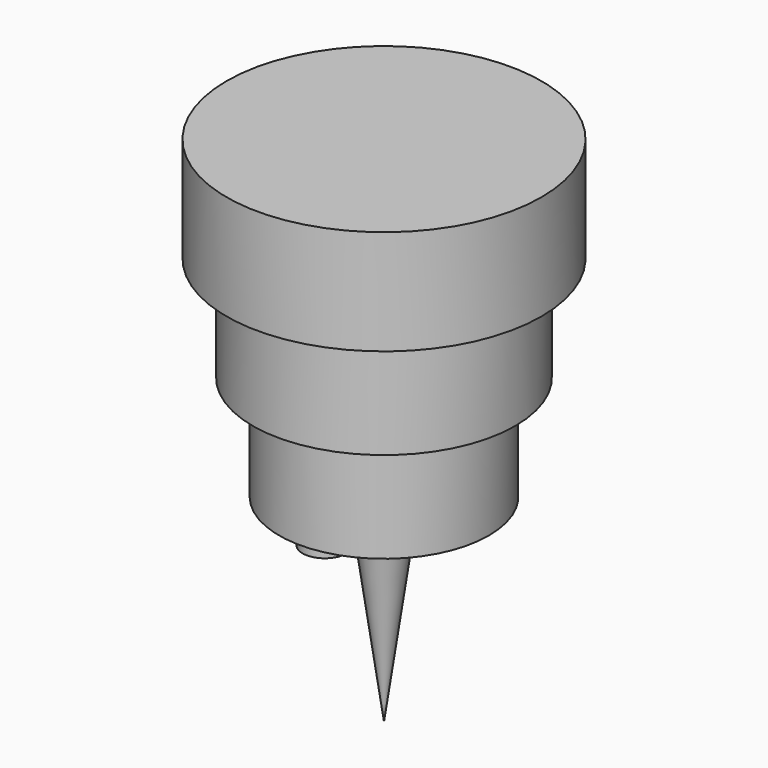
from build123d import *

# Parameters (mm, degrees)
F0_R      = 38.1
F1_DEPTH  = 25.4
F2_R      = 31.75
F3_DEPTH  = 25.4
F4_R      = 25.4
F5_DEPTH  = 50.8
F6_R      = 6.35
F7_DEPTH  = 53.594
F7_FACE_R = 6.35
F10_R     = 5.3624799473
F11_DEPTH = 53.848
F9_R      = 5.3624799473
F12_DEPTH = 53.848


# Not quite as in the source:
# - an extrude whose draft closes it to a point is written as a loft to that point


with BuildPart() as f1:
    # F0 (on Top) → F1 (new body)
    with BuildSketch(Plane.XY):
        Circle(F0_R)
    extrude(amount=F1_DEPTH)

    # F2 (on Top) → F3 (join)
    with BuildSketch(Plane.XY):
        Circle(F2_R)
    extrude(amount=-F3_DEPTH)

    # F4 (on Top) → F5 (join)
    with BuildSketch(Plane.XY):
        Circle(F4_R)
    extrude(amount=-F5_DEPTH)

    # F6 (on Top) → F7 (join)
    with BuildSketch(Plane.XY):
        Circle(F6_R)
    extrude(amount=-F7_DEPTH)

    # F7_face (on face) → F8 section 0
    with BuildSketch(Plane(origin=(0, 0, -53.594), x_dir=(1, 0, 0), z_dir=(0, 0, -1)), mode=Mode.PRIVATE) as f8_s0:
        Circle(F7_FACE_R)
    loft([f8_s0.sketch, Vertex(0, 0, -98.7765977371)], ruled=True)

    # F10 (on Top) → F11 (join)
    with BuildSketch(Plane.XY):
        with Locations((0, 17.3083227128)):
            Circle(F10_R)
    extrude(amount=-F11_DEPTH)

    # F9 (on Top) → F12 (join)
    with BuildSketch(Plane.XY):
        with Locations((0, -17.9224163294)):
            Circle(F9_R)
    extrude(amount=-F12_DEPTH)


solid = f1.part
